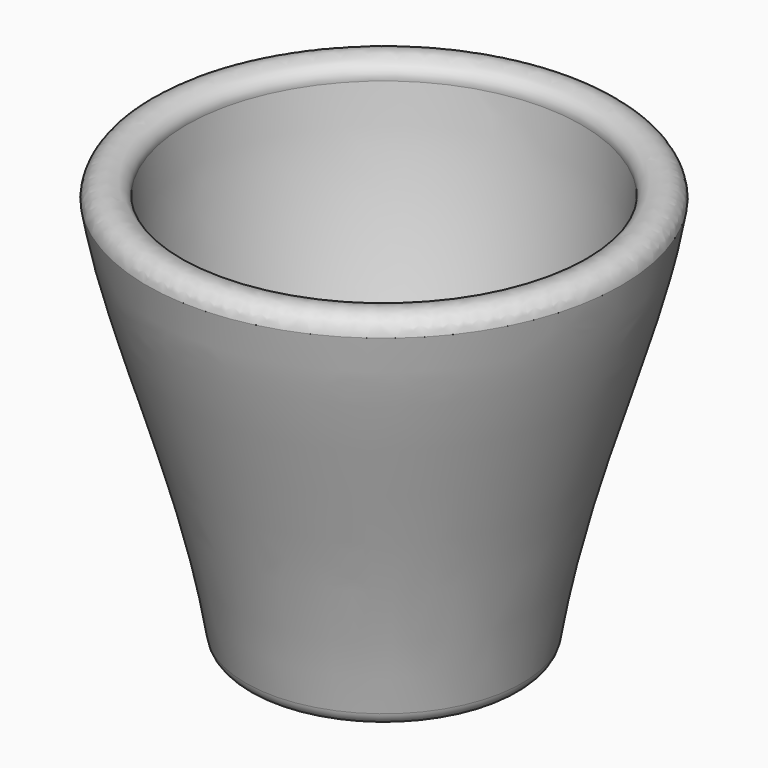
from build123d import *


with BuildPart() as f1:
    # F0 (on Front) → F1 (revolve)
    with BuildSketch(Plane.XZ):
        with BuildLine():
            add(Edge.make_bspline(
                [(-60, 47.3764357992), (-59.1981715925, 54.3134284554), (-49.1629564653, 52.1779667281), (-50, 47.3764357992)],
                knots=[0, 0, 0, 0, 10, 10, 10, 10], degree=3))
            add(Edge.make_bspline(
                [(-60, 47.3764357992), (-55.4738223712, 19.3348543775), (-41.2842135029, -10.1671062354), (-35, -49.2612064975)],
                knots=[0, 0, 0, 0, 100.372548327, 100.372548327, 100.372548327, 100.372548327], degree=3))
            ThreePointArc((-35, -49.2612064975), (-33.5874853172, -51.7190592626), (-30.900831495, -52.6235642008))
            Line((-30.900831495, -52.6235642008), (0, -50.7629300788))
            Line((0, -50.7629300788), (0, -42.7629300788))
            add(Edge.make_bspline(
                [(-27.9523732894, -44.2288875024), (-21.8632061772, -43.3738194628), (-17.4085828413, -42.6430236165), (0, -42.7629300788)],
                knots=[2.9281053207, 2.9281053207, 2.9281053207, 2.9281053207, 30.0507843803, 30.0507843803, 30.0507843803, 30.0507843803], degree=3))
            add(Edge.make_bspline(
                [(-30, -44.5092524641), (-29.2861701407, -44.4149584453), (-28.6097465002, -44.3211987844), (-27.9523732894, -44.2288875024)],
                knots=[0, 0, 0, 0, 2.9281053207, 2.9281053207, 2.9281053207, 2.9281053207], degree=3))
            add(Edge.make_bspline(
                [(-30.2171291126, -42.4791417374), (-30.1386829619, -43.1543106337), (-30.0662089029, -43.8309579045), (-30, -44.5092524641)],
                knots=[91.8520706201, 91.8520706201, 91.8520706201, 91.8520706201, 94.0371187756, 94.0371187756, 94.0371187756, 94.0371187756], degree=3))
            add(Edge.make_bspline(
                [(-50, 47.3764357992), (-47.3655089991, 11.672110508), (-33.514741275, -14.0973136357), (-30.2171291126, -42.4791417374)],
                knots=[0, 0, 0, 0, 91.8520706201, 91.8520706201, 91.8520706201, 91.8520706201], degree=3))
        make_face()
        with BuildLine():
            ThreePointArc((-27.9523732894, -44.2288875024), (-29.4532603476, -43.8309886194), (-30.2171291126, -42.4791417374))
            add(Edge.make_bspline(
                [(-30.2171291126, -42.4791417374), (-30.1386829619, -43.1543106337), (-30.0662089029, -43.8309579045), (-30, -44.5092524641)],
                knots=[91.8520706201, 91.8520706201, 91.8520706201, 91.8520706201, 94.0371187756, 94.0371187756, 94.0371187756, 94.0371187756], degree=3))
            add(Edge.make_bspline(
                [(-30, -44.5092524641), (-29.2861701407, -44.4149584453), (-28.6097465002, -44.3211987844), (-27.9523732894, -44.2288875024)],
                knots=[0, 0, 0, 0, 2.9281053207, 2.9281053207, 2.9281053207, 2.9281053207], degree=3))
        make_face()
    revolve(axis=Axis((0, 0, -1.7270445824), (0, 0, -1)))


solid = f1.part
